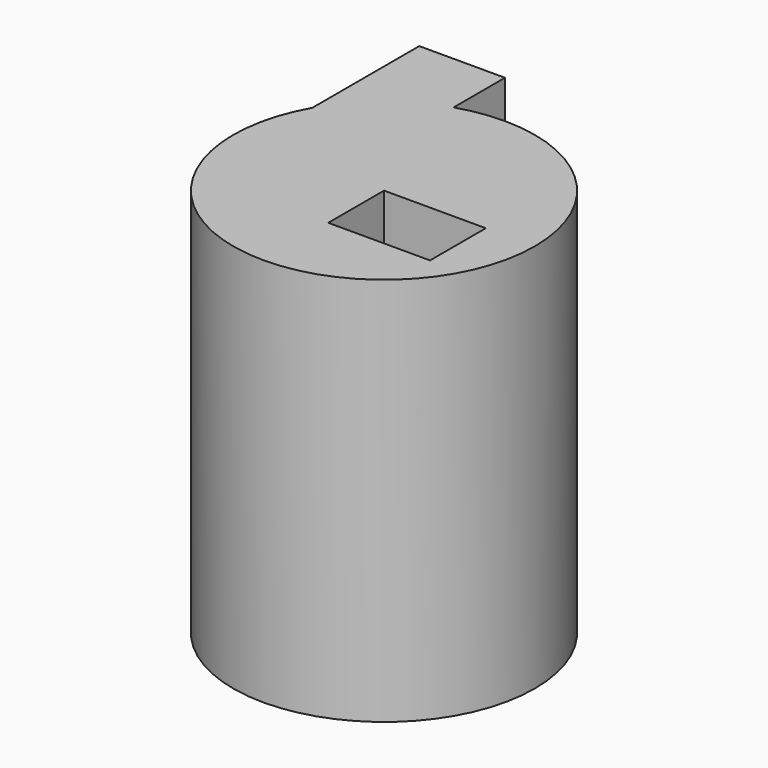
from build123d import *

# Parameters (mm, degrees)
F0_R     = 55.6362832235
F1_DEPTH = 94.234
F3_R     = 55.6362832235
F3_W     = 37.5569760799
F3_H     = 25.7257614285
F4_DEPTH = 49.38980937
F6_DEPTH = 67.5356164575


with BuildPart() as f1:
    # F0 (on Top) → F1 (new body)
    with BuildSketch(Plane.XY):
        Circle(F0_R)
    extrude(amount=F1_DEPTH)

    # F3 (on face) → F4 (join)
    with BuildSketch(Plane.XY.offset(94.234)):
        Circle(F3_R)
        with Locations((18.77848804, -12.8628807142)):
            Rectangle(F3_W, F3_H, mode=Mode.SUBTRACT)
    extrude(amount=F4_DEPTH)

    # F5 (on face) → F6 (join)
    with BuildSketch(Plane.XY.offset(143.62380937)):
        with BuildLine():
            Line((-48.3959540725, 76.7373293638), (-48.3959540725, 27.4449929922))
            ThreePointArc((-48.3959540725, 27.4449929922), (-35.010462285, 43.2396061675), (-16.7768262327, 53.046527808))
            Line((-16.7768262327, 53.046527808), (-16.7768262327, 76.7373293638))
            Line((-16.7768262327, 76.7373293638), (-48.3959540725, 76.7373293638))
        make_face()
    extrude(amount=-F6_DEPTH)


solid = f1.part
